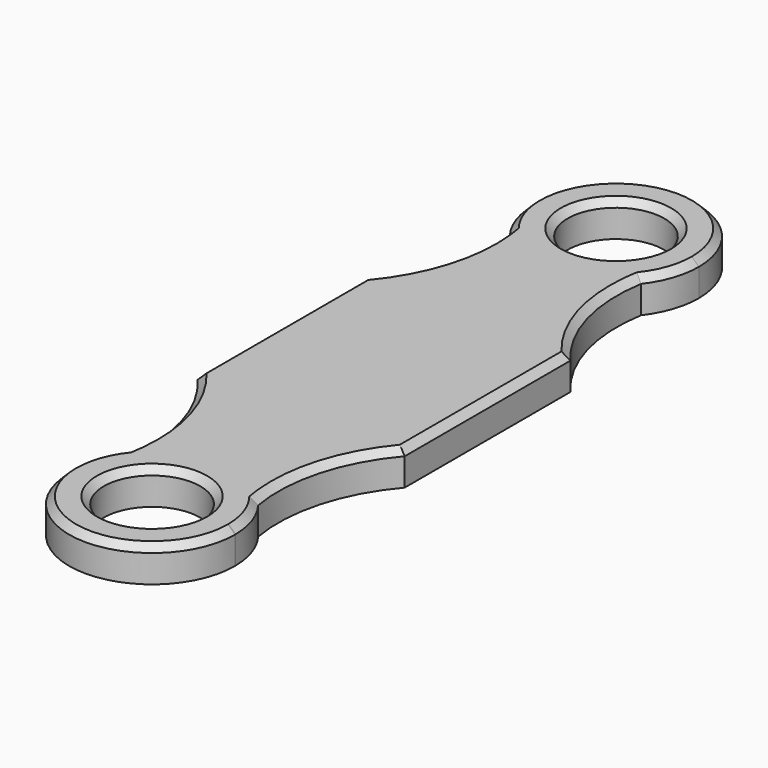
from build123d import *

# Parameters (mm, degrees)
F0_W        = 19.05
F0_H        = 19.05
F0_R        = 0.635
F0_R_2      = 4.445
F1_DEPTH    = 3.175
F2_C1_SIZE  = 0.635
F2_C2_SIZE  = 0.635
F2_C3_SIZE  = 0.635
F2_C4_SIZE  = 0.635
F2_C5_SIZE  = 0.635
F2_C6_SIZE  = 0.635
F2_C7_SIZE  = 0.635
F2_C8_SIZE  = 0.635
F2_C9_SIZE  = 0.6349
F2_C10_SIZE = 0.6349
F3_DEPTH    = 0.635


# Not quite as in the source:
# - a fillet or chamfer is up to 0.001 mm smaller than in the source, because OpenCascade refuses the exact size


with BuildPart() as f1:
    # F0 (on Top) → F1 (new body)
    with BuildSketch(Plane.XY):
        Rectangle(F0_W, F0_H)
        Circle(F0_R, mode=Mode.SUBTRACT)
        with BuildLine():
            Line((9.525, -9.525), (-9.525, -9.525))
            ThreePointArc((-9.525, -9.525), (-6.3836187271, -15.3786997104), (-6.0310725347, -22.012687032))
            ThreePointArc((-6.0310725347, -22.012687032), (0.0350329382, -19.0500805324), (6.0736411029, -22.0683390224))
            ThreePointArc((6.0736411029, -22.0683390224), (6.3936440411, -15.409890989), (9.525, -9.525))
        make_face()
        with BuildLine():
            ThreePointArc((6.0736411029, -22.0683390224), (0.0350329382, -19.0500805324), (-6.0310725347, -22.012687032))
            ThreePointArc((-6.0310725347, -22.012687032), (-6.6363180101, -24.4058987838), (-7.62, -26.67))
            ThreePointArc((-7.62, -26.67), (0, -34.29), (7.62, -26.67))
            ThreePointArc((7.62, -26.67), (7.619882327, -26.6276523681), (7.6195293118, -26.5853060441))
            ThreePointArc((7.6195293118, -26.5853060441), (6.6686101992, -24.3877327559), (6.0736411029, -22.0683390224))
        make_face()
        with Locations((0, -26.67)):
            Circle(F0_R_2, mode=Mode.SUBTRACT)
        with BuildLine():
            ThreePointArc((-7.62, -26.67), (-6.6363180101, -24.4058987838), (-6.0310725347, -22.012687032))
            ThreePointArc((-6.0310725347, -22.012687032), (-7.2118365454, -24.2095501137), (-7.62, -26.67))
        make_face()
        with BuildLine():
            ThreePointArc((7.6195293118, -26.5853060441), (7.2094713239, -24.202628275), (6.0736411029, -22.0683390224))
            ThreePointArc((6.0736411029, -22.0683390224), (6.6686101992, -24.3877327559), (7.6195293118, -26.5853060441))
        make_face()
        with BuildLine():
            ThreePointArc((-6.0736411029, 22.0683390224), (-6.3936440411, 15.409890989), (-9.525, 9.525))
            Line((-9.525, 9.525), (9.525, 9.525))
            ThreePointArc((9.525, 9.525), (6.3836187271, 15.3786997104), (6.0310725347, 22.012687032))
            ThreePointArc((6.0310725347, 22.012687032), (-0.0350329382, 19.0500805324), (-6.0736411029, 22.0683390224))
        make_face()
        with BuildLine():
            ThreePointArc((-7.6195293118, 26.5853060441), (-6.6686101992, 24.3877327559), (-6.0736411029, 22.0683390224))
            ThreePointArc((-6.0736411029, 22.0683390224), (-0.0350329382, 19.0500805324), (6.0310725347, 22.012687032))
            ThreePointArc((6.0310725347, 22.012687032), (6.6363180101, 24.4058987838), (7.62, 26.67))
            ThreePointArc((7.62, 26.67), (-0.0423476319, 34.289882327), (-7.6195293118, 26.5853060441))
        make_face()
        with Locations((0, 26.67)):
            Circle(F0_R_2, mode=Mode.SUBTRACT)
        with BuildLine():
            ThreePointArc((-7.6195293118, 26.5853060441), (-7.2094713239, 24.202628275), (-6.0736411029, 22.0683390224))
            ThreePointArc((-6.0736411029, 22.0683390224), (-6.6686101992, 24.3877327559), (-7.6195293118, 26.5853060441))
        make_face()
        with BuildLine():
            ThreePointArc((7.62, 26.67), (6.6363180101, 24.4058987838), (6.0310725347, 22.012687032))
            ThreePointArc((6.0310725347, 22.012687032), (7.2118365454, 24.2095501137), (7.62, 26.67))
        make_face()
        Circle(F0_R)
    extrude(amount=F1_DEPTH)

    # F2: chamfer of 0.635 on 10 edges, made by hand

    # F2_c1
    f2_c1_edges = [f1.edges().sort_by_distance(p)[0] for p in [
        (-9.525, 0, 3.175),
    ]]
    chamfer(f2_c1_edges, length=F2_C1_SIZE)

    # F2_c2
    f2_c2_edges = [f1.edges().sort_by_distance(p)[0] for p in [
        (-6.2554888364, -15.867774564, 3.175),
    ]]
    chamfer(f2_c2_edges, length=F2_C2_SIZE)

    # F2_c3
    f2_c3_edges = [f1.edges().sort_by_distance(p)[0] for p in [
        (6.3936440411, -15.409890989, 3.175),
    ]]
    chamfer(f2_c3_edges, length=F2_C3_SIZE)

    # F2_c4
    f2_c4_edges = [f1.edges().sort_by_distance(p)[0] for p in [
        (9.525, 0.4748240758, 3.175),
    ]]
    chamfer(f2_c4_edges, length=F2_C4_SIZE)

    # F2_c5
    f2_c5_edges = [f1.edges().sort_by_distance(p)[0] for p in [
        (6.2554888364, 15.867774564, 3.175),
    ]]
    chamfer(f2_c5_edges, length=F2_C5_SIZE)

    # F2_c6
    f2_c6_edges = [f1.edges().sort_by_distance(p)[0] for p in [
        (-6.2671958343, 15.9012829536, 3.175),
    ]]
    chamfer(f2_c6_edges, length=F2_C6_SIZE)

    # F2_c7
    f2_c7_edges = [f1.edges().sort_by_distance(p)[0] for p in [
        (-4.445, -26.67, 3.175),
    ]]
    chamfer(f2_c7_edges, length=F2_C7_SIZE)

    # F2_c8
    f2_c8_edges = [f1.edges().sort_by_distance(p)[0] for p in [
        (-4.445, 26.67, 3.175),
    ]]
    chamfer(f2_c8_edges, length=F2_C8_SIZE)

    # F2_c9 (size 0.635 in the source; OpenCascade refuses exactly that, so slightly less here)
    f2_c9_edges = [f1.edges().sort_by_distance(p)[0] for p in [
        (-0.0350329382, -34.2899194676, 3.175),
    ]]
    chamfer(f2_c9_edges, length=F2_C9_SIZE)

    # F2_c10 (size 0.635 in the source; OpenCascade refuses exactly that, so slightly less here)
    f2_c10_edges = [f1.edges().sort_by_distance(p)[0] for p in [
        (0.0350329382, 34.2899194676, 3.175),
    ]]
    chamfer(f2_c10_edges, length=F2_C10_SIZE)

    # F0 (on Top) → F3 (cut)
    with BuildSketch(Plane.XY):
        Circle(F0_R)
    extrude(amount=F3_DEPTH, mode=Mode.SUBTRACT)


solid = f1.part
